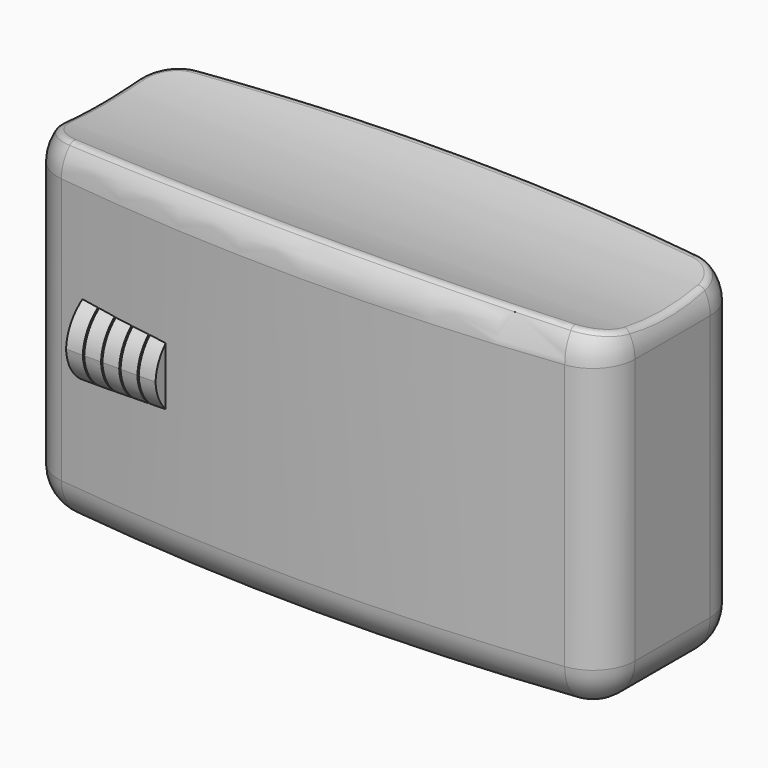
from build123d import *

# Parameters (mm, degrees)
F1_DEPTH       = 25
F2_R           = 3
F3_R           = 25
F4_DEPTH       = 48.9
F5_W           = 35.273212415
F5_H           = 6.729037715
F6_DEPTH       = 21.7
F7_W           = 3
F7_H           = 7
F8_DEPTH       = 25
F9_R           = 0.5
F11_START      = 5.3
F10_W          = 1.2
F10_H          = 6
F11_DEPTH      = 2.7
F10_W_2        = 1.2000006843
F12_T1_DEPTH   = 17.0034806293
F12_2_T1_DEPTH = 17.0034806293
F12_3_T1_DEPTH = 17.0034806293
F12_4_T1_DEPTH = 17.0034806293
F12_5_T1_DEPTH = 17.0034813136
F13_R          = 2.5
F14_DEPTH      = 22.5
F15_W          = 3
F15_H          = 1.5
F16_DEPTH      = 2
F17_W          = 3
F17_H          = 1.5
F18_DEPTH      = 2
F19_W          = 4
F19_H          = 1.5
F20_DEPTH      = 1.5
F21_W          = 4
F21_H          = 1.5
F22_DEPTH      = 1.5
F23_W          = 4
F23_H          = 1.5
F24_DEPTH      = 1.5
F25_W          = 4
F25_H          = 1.5
F26_DEPTH      = 1.5


# Not quite as in the source:
# - a fillet or chamfer that OpenCascade refuses, or shapes differently, is made with other operations: its cross-section is extruded or revolved along the edge and cut away or added


with BuildPart() as f1:
    # F0 (on Top) → F1 (new body)
    with BuildSketch(Plane.XY):
        with BuildLine():
            ThreePointArc((20.6366062075, 6), (0, 7.4263466013), (-20.6366062075, 6))
            Line((-20.6366062075, 6), (-20.6366062075, -6))
            ThreePointArc((-20.6366062075, -6), (0, -7.4263466013), (20.6366062075, -6))
            Line((20.6366062075, -6), (20.6366062075, 6))
        make_face()
    extrude(amount=F1_DEPTH)

    # F2
    f2_edges = [f1.edges().sort_by_distance(p)[0] for p in [
        (-20.636606, 6, 12.5),
        (-20.636606, -6, 12.5),
        (20.636606, 6, 12.5),
        (20.636606, -6, 12.5),
        (0, 7.426347, 0),
        (0, -7.426347, 0),
        (-20.636606, 0, 0),
        (20.636606, 0, 0),
        (0, -7.426347, 25),
        (20.636606, 0, 25),
        (0, 7.426347, 25),
        (-20.636606, 0, 25),
    ]]
    fillet(f2_edges, radius=F2_R)

    # F3 (on face) → F4 (cut)
    with BuildSketch(Plane.YZ.offset(20.6366062075)):
        with Locations((0, 48.5)):
            Circle(F3_R)
    extrude(amount=-F4_DEPTH, mode=Mode.SUBTRACT)

    # F5 (on face) → F6 (cut)
    with BuildSketch(Plane(origin=(0, 0, 0), x_dir=(1, 0, 0), z_dir=(0, 0, -1))):
        Rectangle(F5_W, F5_H)
    extrude(amount=-F6_DEPTH, mode=Mode.SUBTRACT)

    # F7 (on face) → F8 (cut)
    with BuildSketch(Plane(origin=(-20.6366062075, 0, 0), x_dir=(0, -1, 0), z_dir=(-1, 0, 0))):
        with Locations((0, 7.0144929923)):
            Rectangle(F7_W, F7_H)
    extrude(amount=-F8_DEPTH, mode=Mode.SUBTRACT)

    # F9
    f9_edges = [f1.edges().sort_by_distance(p)[0] for p in [
        (19.37767, -4.812689, 23.967613),
        (20.234682, 0, 23.5),
        (19.37767, 4.812689, 23.967613),
        (0, 6.333682, 24.315615),
        (-19.37767, 4.812689, 23.967613),
        (-20.234682, 0, 23.5),
        (-19.37767, -4.812689, 23.967613),
        (0, -6.333682, 24.315615),
    ]]
    fillet(f9_edges, radius=F9_R)

    # F13 (on Top) → F14 (cut)
    with BuildSketch(Plane.XY):
        with Locations((-11.2689465519, 0)):
            Circle(F13_R)
        Circle(F13_R)
        with Locations((11.2689465519, 0)):
            Circle(F13_R)
    extrude(amount=F14_DEPTH, mode=Mode.SUBTRACT)

    # F15 (on face) → F16 (cut)
    with BuildSketch(Plane.XZ.offset(-3.3645188575)):
        with Locations((-13.1366062075, 20.95)):
            Rectangle(F15_W, F15_H)
        with Locations((13.1366062075, 20.95)):
            Rectangle(F15_W, F15_H)
    extrude(amount=-F16_DEPTH, mode=Mode.SUBTRACT)

    # F17 (on face) → F18 (cut)
    with BuildSketch(Plane(origin=(0, -3.3645188575, 0), x_dir=(-1, 0, 0), z_dir=(0, 1, 0))):
        with Locations((-13.1777257323, 20.95)):
            Rectangle(F17_W, F17_H)
        with Locations((13.1777257323, 20.95)):
            Rectangle(F17_W, F17_H)
    extrude(amount=-F18_DEPTH, mode=Mode.SUBTRACT)

    # F19 (on face) → F20 (cut)
    with BuildSketch(Plane(origin=(17.6366062075, 0, 0), x_dir=(0, -1, 0), z_dir=(-1, 0, 0))):
        with Locations((0.0004811425, 1.75)):
            Rectangle(F19_W, F19_H)
    extrude(amount=-F20_DEPTH, mode=Mode.SUBTRACT)

    # F21 (on face) → F22 (cut)
    with BuildSketch(Plane.YZ.offset(-17.6366062075)):
        with Locations((-0.0004811425, 1.75)):
            Rectangle(F21_W, F21_H)
    extrude(amount=-F22_DEPTH, mode=Mode.SUBTRACT)

    # F23 (on face) → F24 (cut)
    with BuildSketch(Plane.XZ.offset(-3.3645188575)):
        with Locations((0, 1.75)):
            Rectangle(F23_W, F23_H)
    extrude(amount=-F24_DEPTH, mode=Mode.SUBTRACT)

    # F25 (on face) → F26 (cut)
    with BuildSketch(Plane(origin=(0, -3.3645188575, 0), x_dir=(-1, 0, 0), z_dir=(0, 1, 0))):
        with Locations((0, 1.75)):
            Rectangle(F25_W, F25_H)
    extrude(amount=-F26_DEPTH, mode=Mode.SUBTRACT)


with BuildPart() as f11:
    # F10 (on Front) → F11 (new body)
    with BuildSketch(Plane.XZ.offset(F11_START)):
        with Locations((-14.4426309329, 12.5)):
            Rectangle(F10_W, F10_H)
    extrude(amount=F11_DEPTH)

    # F12: fillet of radius 3.2 on 2 edges, made by hand

    # F12_s2 → F12_t1 (cut)
    with BuildSketch(Plane.YZ.offset(-22.9443712476)):
        with BuildLine():
            ThreePointArc((-5.3, 15.5), (-7.2331050121, 14.4177648432), (-8, 12.3393038741))
            Line((-8, 12.3393038741), (-8, 15.5))
            Line((-8, 15.5), (-5.3, 15.5))
        make_face()
        with BuildLine():
            ThreePointArc((-5.3, 9.5), (-7.2331050121, 10.5822351568), (-8, 12.6606961259))
            Line((-8, 12.6606961259), (-8, 9.5))
            Line((-8, 9.5), (-5.3, 9.5))
        make_face()
    extrude(amount=F12_T1_DEPTH, mode=Mode.SUBTRACT)


with BuildPart() as f11b:
    # F10 (on Front) → F11, piece 2 (new body)
    with BuildSketch(Plane.XZ.offset(F11_START)):
        with Locations((-13.1426309329, 12.5)):
            Rectangle(F10_W, F10_H)
    extrude(amount=F11_DEPTH)

    # F12#2: fillet of radius 3.2 on 2 edges, made by hand

    # F12_2_s2 → F12_2_t1 (cut)
    with BuildSketch(Plane.YZ.offset(-21.6443712476)):
        with BuildLine():
            ThreePointArc((-5.3, 15.5), (-7.2331050121, 14.4177648432), (-8, 12.3393038741))
            Line((-8, 12.3393038741), (-8, 15.5))
            Line((-8, 15.5), (-5.3, 15.5))
        make_face()
        with BuildLine():
            ThreePointArc((-5.3, 9.5), (-7.2331050121, 10.5822351568), (-8, 12.6606961259))
            Line((-8, 12.6606961259), (-8, 9.5))
            Line((-8, 9.5), (-5.3, 9.5))
        make_face()
    extrude(amount=F12_2_T1_DEPTH, mode=Mode.SUBTRACT)


with BuildPart() as f11c:
    # F10 (on Front) → F11, piece 3 (new body)
    with BuildSketch(Plane.XZ.offset(F11_START)):
        with Locations((-11.8426309329, 12.5)):
            Rectangle(F10_W, F10_H)
    extrude(amount=F11_DEPTH)

    # F12#3: fillet of radius 3.2 on 2 edges, made by hand

    # F12_3_s2 → F12_3_t1 (cut)
    with BuildSketch(Plane.YZ.offset(-20.3443712476)):
        with BuildLine():
            ThreePointArc((-5.3, 15.5), (-7.2331050121, 14.4177648432), (-8, 12.3393038741))
            Line((-8, 12.3393038741), (-8, 15.5))
            Line((-8, 15.5), (-5.3, 15.5))
        make_face()
        with BuildLine():
            ThreePointArc((-5.3, 9.5), (-7.2331050121, 10.5822351568), (-8, 12.6606961259))
            Line((-8, 12.6606961259), (-8, 9.5))
            Line((-8, 9.5), (-5.3, 9.5))
        make_face()
    extrude(amount=F12_3_T1_DEPTH, mode=Mode.SUBTRACT)


with BuildPart() as f11d:
    # F10 (on Front) → F11, piece 4 (new body)
    with BuildSketch(Plane.XZ.offset(F11_START)):
        Polygon((-9.9426309329, 15.5), (-11.1426309329, 15.5), (-11.1426309329, 9.5), (-9.9426309329, 9.5), (-9.9426309329, 11.9), (-9.9426309329, 13), align=None)
    extrude(amount=F11_DEPTH)

    # F12#4: fillet of radius 3.2 on 2 edges, made by hand

    # F12_4_s2 → F12_4_t1 (cut)
    with BuildSketch(Plane.YZ.offset(-19.0443712476)):
        with BuildLine():
            ThreePointArc((-5.3, 15.5), (-7.2331050121, 14.4177648432), (-8, 12.3393038741))
            Line((-8, 12.3393038741), (-8, 15.5))
            Line((-8, 15.5), (-5.3, 15.5))
        make_face()
        with BuildLine():
            ThreePointArc((-8, 12.6606961259), (-7.2331050121, 10.5822351568), (-5.3, 9.5))
            Line((-5.3, 9.5), (-8, 9.5))
            Line((-8, 9.5), (-8, 12.6606961259))
        make_face()
    extrude(amount=F12_4_T1_DEPTH, mode=Mode.SUBTRACT)


with BuildPart() as f11e:
    # F10 (on Front) → F11, piece 5 (new body)
    with BuildSketch(Plane.XZ.offset(F11_START)):
        with Locations((-15.7426312751, 12.5)):
            Rectangle(F10_W_2, F10_H)
    extrude(amount=F11_DEPTH)

    # F12#5: fillet of radius 3.2 on 2 edges, made by hand

    # F12_5_s2 → F12_5_t1 (cut)
    with BuildSketch(Plane.YZ.offset(-24.2443719319)):
        with BuildLine():
            ThreePointArc((-5.3, 15.5), (-7.2331050121, 14.4177648432), (-8, 12.3393038741))
            Line((-8, 12.3393038741), (-8, 15.5))
            Line((-8, 15.5), (-5.3, 15.5))
        make_face()
        with BuildLine():
            ThreePointArc((-5.3, 9.5), (-7.2331050121, 10.5822351568), (-8, 12.6606961259))
            Line((-8, 12.6606961259), (-8, 9.5))
            Line((-8, 9.5), (-5.3, 9.5))
        make_face()
    extrude(amount=F12_5_T1_DEPTH, mode=Mode.SUBTRACT)


solid = Compound([f1.part, f11.part, f11b.part, f11c.part, f11d.part, f11e.part])
